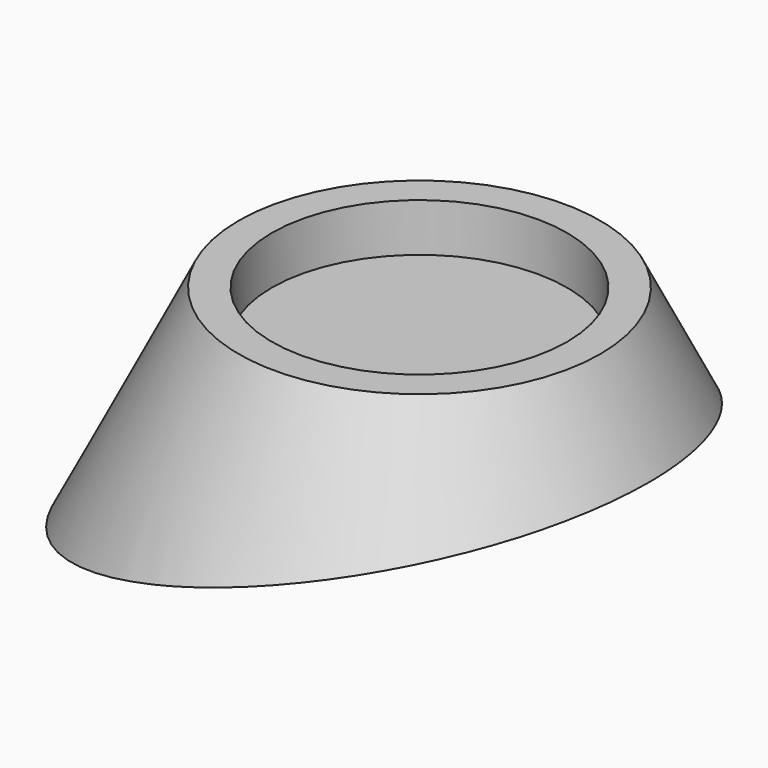
from build123d import *

# Parameters (mm, degrees)
F0_R     = 12.5
F1_DEPTH = 10
F2_SIZE2 = 9.99999
F2_SIZE  = 4.99999
F4_DEPTH = 12.5
F5_R     = 6.125
F6_DEPTH = 2


# Not quite as in the source:
# - a fillet or chamfer is up to 0.001 mm smaller than in the source, because OpenCascade refuses the exact size


with BuildPart() as f1:
    # F0 (on Top) → F1 (new body)
    with BuildSketch(Plane.XY):
        Circle(F0_R)
    extrude(amount=F1_DEPTH)

    # F2 (size 5 and 10 in the source; OpenCascade refuses exactly that, so slightly less here)
    f2_edges = [f1.edges().sort_by_distance(p)[0] for p in [
        (-12.5, 0, 10),
    ]]
    f2_side = f1.faces().sort_by_distance((0, 0, 10))[0]
    chamfer(f2_edges, length=F2_SIZE, length2=F2_SIZE2, reference=f2_side)

    # F3 (on Front) → F4 (cut, symmetric)
    with BuildSketch(Plane.XZ):
        Polygon((11.7184263772, 6.5591478468), (-12.7606466413, 0), (-7.277042605, -3.8485343102), (16.1768086255, -2.4198731408), align=None)
    extrude(amount=F4_DEPTH, both=True, mode=Mode.SUBTRACT)

    # F5 (on face) → F6 (cut)
    with BuildSketch(Plane.XY.offset(10)):
        Circle(F5_R)
    extrude(amount=-F6_DEPTH, mode=Mode.SUBTRACT)


solid = f1.part
